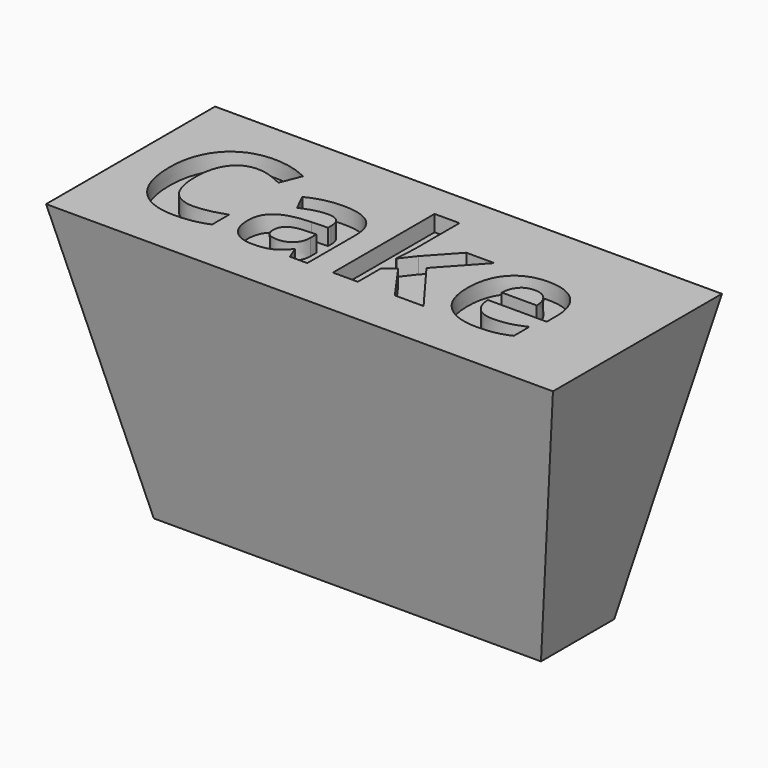
from build123d import *

# Parameters (mm, degrees)
F0_W         = 1828.8
F0_H         = 762
F1_DEPTH     = 1016
F1_TAPER     = 12
F2_TEXT_SIZE = 603.4378583233
F3_DEPTH     = 58.42


# Not quite as in the source:
# - Text() gives the source's letters only with a copy of the font that has no kerning and outlines rounded to 1/6400 em; it was checked with that copy


with BuildPart() as f1:
    # F0 (on Top) → F1 (new body)
    with BuildSketch(Plane.XY):
        Rectangle(F0_W, F0_H)
    extrude(amount=-F1_DEPTH, taper=F1_TAPER)

    # F2 (on face) → F3 (cut)
    with BuildSketch(Plane.XY):
        with Locations((-818.4124231339, -202.5520652533)):
            Text('Cake', F2_TEXT_SIZE, font='Open Sans', font_style=FontStyle.BOLD, text_align=(TextAlign.LEFT, TextAlign.BOTTOM))
    extrude(amount=-F3_DEPTH, mode=Mode.SUBTRACT)


solid = f1.part
